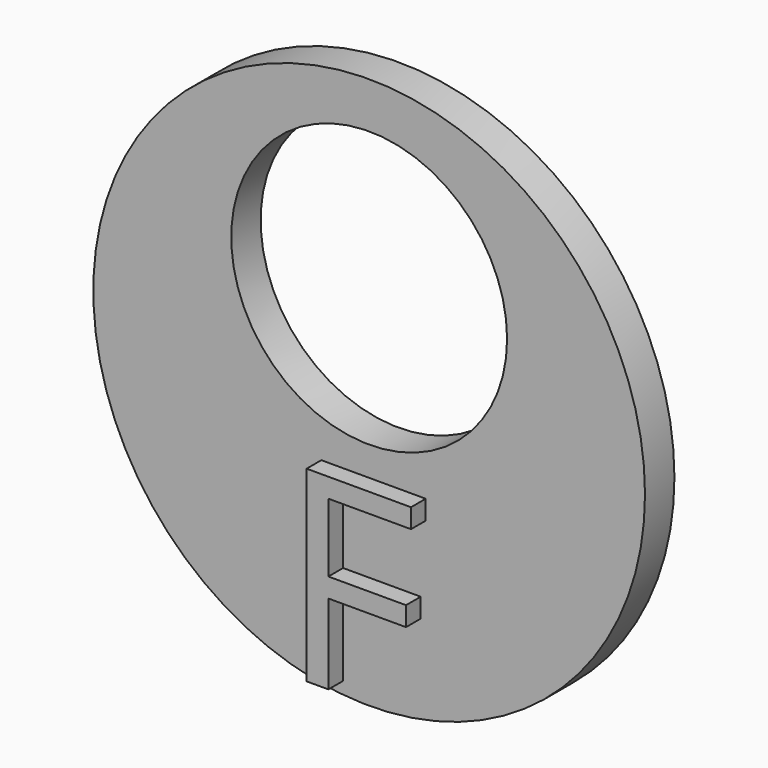
from build123d import *

# Parameters (mm, degrees)
F0_R         = 15
F0_R_2       = 7.5
F1_DEPTH     = 2
F2_TEXT_SIZE = 14.2618384401
F3_DEPTH     = 1


# Not quite as in the source:
# - Text() gives the source's letters only with a copy of the font that has no kerning and outlines rounded to 1/6400 em; it was checked with that copy


with BuildPart() as f1:
    # F0 (on Front) → F1 (new body)
    with BuildSketch(Plane.XZ):
        Circle(F0_R)
        with Locations((0, 5)):
            Circle(F0_R_2, mode=Mode.SUBTRACT)
    extrude(amount=F1_DEPTH)

    # F2 (on face) → F3 (join)
    with BuildSketch(Plane.XZ.offset(2)):
        with Locations((-4, -14.2685236769)):
            Text('F', F2_TEXT_SIZE, font='Open Sans', text_align=(TextAlign.LEFT, TextAlign.BOTTOM))
    extrude(amount=F3_DEPTH)


solid = f1.part
